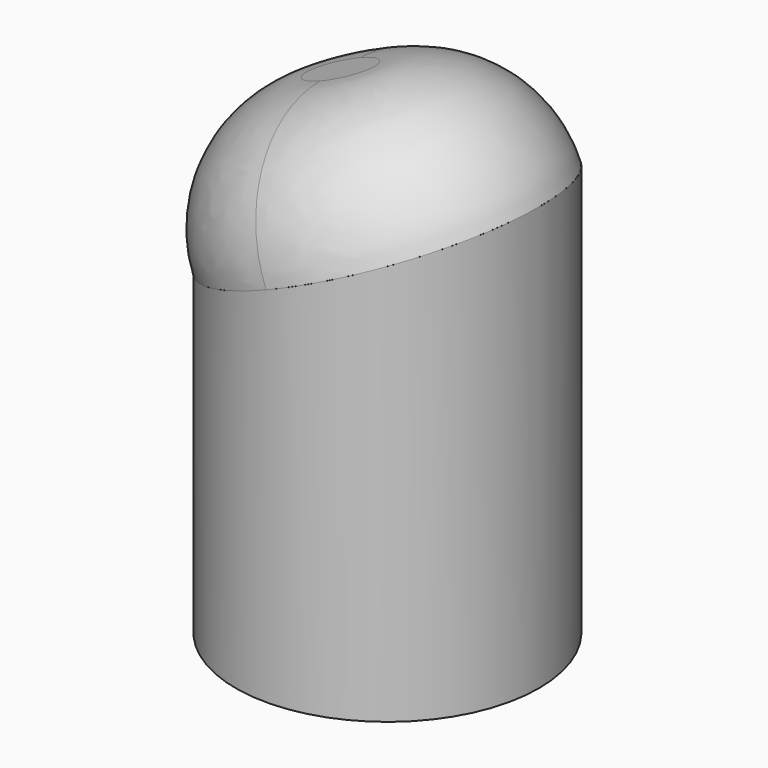
from build123d import *

# Parameters (mm, degrees)
F0_R     = 2.4
F1_DEPTH = 10
F3_DEPTH = 4
F5_DEPTH = 2
F6_R     = 1.9999


# Not quite as in the source:
# - a fillet or chamfer is up to 0.001 mm smaller than in the source, because OpenCascade refuses the exact size
# - a feature names something its author has since deleted; it is built from what else it names


with BuildPart() as f1:
    # F0 (on Top) → F1 (new body)
    with BuildSketch(Plane.XY):
        Circle(F0_R)
    extrude(amount=F1_DEPTH)

    # F2 (on Front) → F3 (cut, symmetric)
    with BuildSketch(Plane.XZ):
        Polygon((-2.5, 10.5), (-2.5, 4.75), (2.5, 6.75), (2.5, 10.5), align=None)
    extrude(amount=F3_DEPTH, both=True, mode=Mode.SUBTRACT)

    # F4 (on face) → F5 (join)
    with BuildSketch(Plane(origin=(-1.9827586207, 0, 4.9568965517), x_dir=(0.9284766909, 0, 0.3713906764), z_dir=(-0.3713906764, 0, 0.9284766909))):
        with BuildLine():
            add(Edge.make_bspline(
                [(2.135496578, 2.4), (4.7203754965, 2.3999998246), (4.7203754965, 0)],
                knots=[7.8915744057, 7.8915744057, 7.8915744057, 9.4247779608, 9.4247779608, 9.4247779608], degree=2, weights=[0.8038475615, 0.6339746132, 1]))
            add(Edge.make_bspline(
                [(2.1354967017, -2.4), (1.4428802648, -2.4000000778), (0.8430568353, -2.0784609691), (-3.0342618258, 0), (0.8430568353, 2.0784609691), (1.4428802074, 2.400000047), (2.135496578, 2.4)],
                knots=[4.6747961621, 4.6747961621, 4.6747961621, 5.235987756, 5.235987756, 7.3303828584, 7.3303828584, 7.8915744057, 7.8915744057, 7.8915744057], degree=2, weights=[0.8038475512, 0.8660253757, 1, 0.5, 1, 0.8660253868, 0.8038475615]))
            add(Edge.make_bspline(
                [(4.7203754965, 0), (4.7203754965, -2.3999997097), (2.1354967017, -2.4)],
                knots=[3.1415926536, 3.1415926536, 3.1415926536, 4.6747961621, 4.6747961621, 4.6747961621], degree=2, weights=[1, 0.6339746243, 0.8038475512]))
        make_face()
    extrude(amount=F5_DEPTH)

    # F6 (radius 2 in the source; OpenCascade refuses exactly that, so slightly less here)
    f6_edges = [f1.edges().sort_by_distance(p)[0] for p in [
        (1.029171, -1.618698, 8.315734),
        (-3.142781, 0, 6.646953),
        (1.029171, 1.618698, 8.315734),
    ]]
    fillet(f6_edges, radius=F6_R)


solid = f1.part
